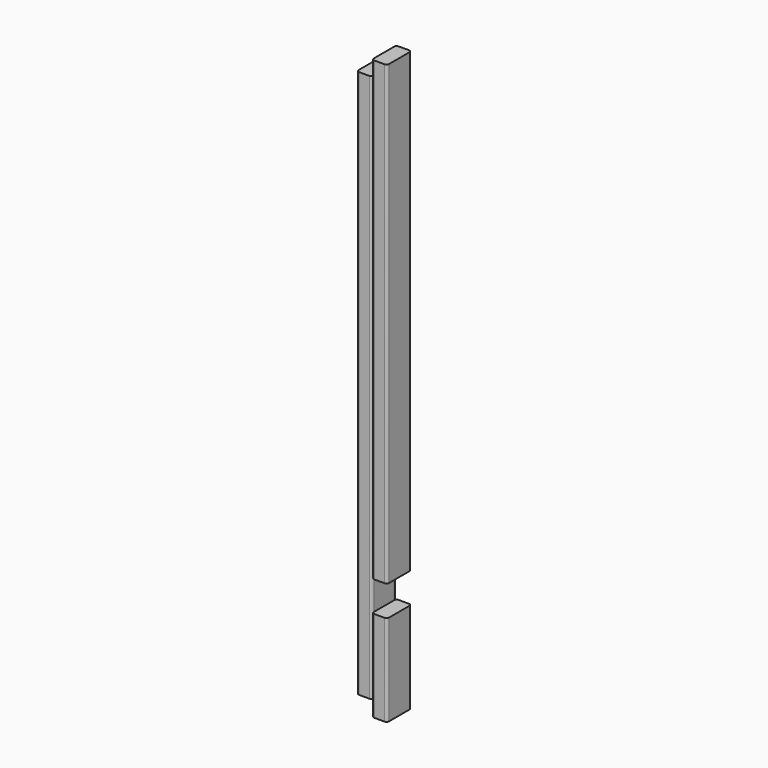
from build123d import *

# Parameters (mm, degrees)
F1_DEPTH = 723.9
F2_DEPTH = 704.85
F3_DEPTH = 19.05
F4_W     = 3.1496
F4_H     = 38.1
F4_W_2   = 12.7508
F5_DEPTH = 38.101


# Not quite as in the source:
# - a feature names something its author has since deleted; it is built from what else it names


with BuildPart() as f1:
    # F0 (on Top) → F1 (new body)
    with BuildSketch(Plane.XY):
        with BuildLine():
            Line((19.05, 34.9504), (19.05, 3.1496))
            ThreePointArc((19.05, 3.1496), (19.972496482, 0.922496482), (22.1996, 0))
            Line((22.1996, 0), (34.9504, 0))
            ThreePointArc((34.9504, 0), (37.177503518, 0.922496482), (38.1, 3.1496))
            Line((38.1, 3.1496), (38.1, 34.9504))
            ThreePointArc((38.1, 34.9504), (37.177503518, 37.177503518), (34.9504, 38.1))
            Line((34.9504, 38.1), (22.1996, 38.1))
            ThreePointArc((22.1996, 38.1), (19.972496482, 37.177503518), (19.05, 34.9504))
        make_face()
    extrude(amount=F1_DEPTH)

    # F0 (on Top) → F2 (join)
    with BuildSketch(Plane.XY):
        with BuildLine():
            ThreePointArc((0, 3.1496), (0.922496482, 0.922496482), (3.1496, 0))
            Line((3.1496, 0), (15.9004, 0))
            ThreePointArc((15.9004, 0), (18.127503518, 0.922496482), (19.05, 3.1496))
            Line((19.05, 3.1496), (19.05, 34.9504))
            ThreePointArc((19.05, 34.9504), (18.127503518, 37.177503518), (15.9004, 38.1))
            Line((15.9004, 38.1), (3.1496, 38.1))
            ThreePointArc((3.1496, 38.1), (0.922496482, 37.177503518), (0, 34.9504))
            Line((0, 34.9504), (0, 3.1496))
        make_face()
        with BuildLine():
            Line((19.05, 34.9504), (19.05, 3.1496))
            ThreePointArc((19.05, 3.1496), (19.972496482, 0.922496482), (22.1996, 0))
            Line((22.1996, 0), (34.9504, 0))
            ThreePointArc((34.9504, 0), (37.177503518, 0.922496482), (38.1, 3.1496))
            Line((38.1, 3.1496), (38.1, 34.9504))
            ThreePointArc((38.1, 34.9504), (37.177503518, 37.177503518), (34.9504, 38.1))
            Line((34.9504, 38.1), (22.1996, 38.1))
            ThreePointArc((22.1996, 38.1), (19.972496482, 37.177503518), (19.05, 34.9504))
        make_face()
    extrude(amount=F2_DEPTH)

    # F0 (on Top) → F3 (cut)
    with BuildSketch(Plane.XY):
        with BuildLine():
            ThreePointArc((0, 3.1496), (0.922496482, 0.922496482), (3.1496, 0))
            Line((3.1496, 0), (15.9004, 0))
            ThreePointArc((15.9004, 0), (18.127503518, 0.922496482), (19.05, 3.1496))
            Line((19.05, 3.1496), (19.05, 34.9504))
            ThreePointArc((19.05, 34.9504), (18.127503518, 37.177503518), (15.9004, 38.1))
            Line((15.9004, 38.1), (3.1496, 38.1))
            ThreePointArc((3.1496, 38.1), (0.922496482, 37.177503518), (0, 34.9504))
            Line((0, 34.9504), (0, 3.1496))
        make_face()
    extrude(amount=F3_DEPTH, mode=Mode.SUBTRACT)

    # F4 (on face) → F5 (cut, through all)
    with BuildSketch(Plane.XZ):
        with Locations((36.5252, 133.35)):
            Rectangle(F4_W, F4_H)
        with Locations((28.575, 133.35)):
            Rectangle(F4_W_2, F4_H)
        with Locations((20.6248, 133.35)):
            Rectangle(F4_W, F4_H)
    extrude(amount=-F5_DEPTH, mode=Mode.SUBTRACT)


solid = f1.part
